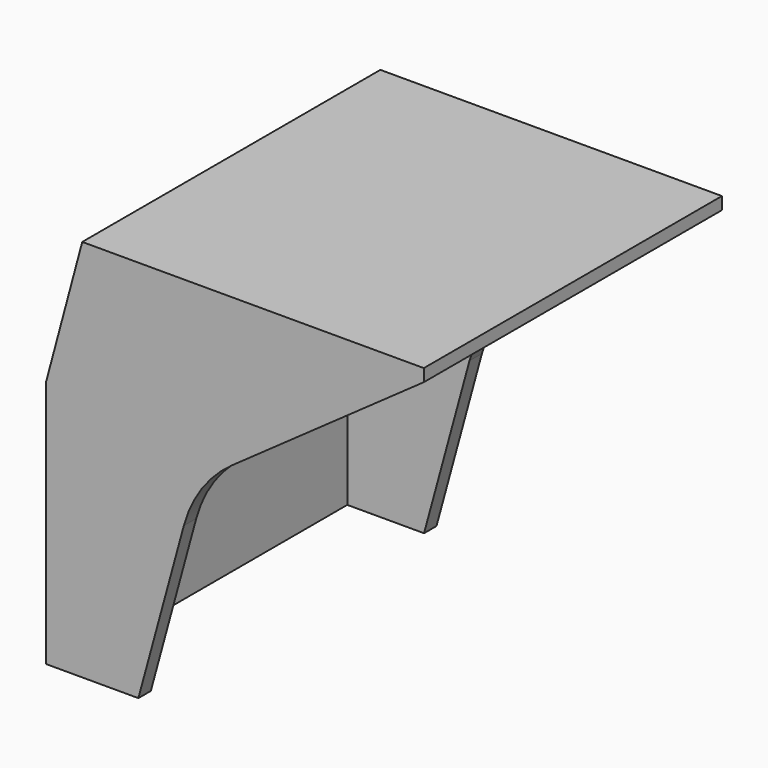
from build123d import *

# Parameters (mm, degrees)
F1_DEPTH  = 120
F2_W      = 85.2778990954
F2_H      = 80
F3_DEPTH  = 98
F6_DEPTH  = 80
F7_W      = 105
F7_H      = 80
F8_DEPTH  = 120
F9_DEPTH  = 15
F10_DEPTH = 30
F11_DEPTH = 15


with BuildPart() as f1:
    # F0 (on Front) → F1 (new body)
    with BuildSketch(Plane.XZ):
        with BuildLine():
            Line((0, 80), (0, 0))
            Line((0, 0), (29.7221009046, 0))
            Line((29.7221009046, 0), (44.3633417849, 53.6774845415))
            ThreePointArc((44.3633417849, 53.6774845415), (50.1903143406, 66.0986305535), (59.871849565, 75.8200683645))
            Line((59.871849565, 75.8200683645), (121.6468570296, 119.466662183))
            Line((121.6468570296, 119.466662183), (121.6468570296, 123.466662183))
            Line((121.6468570296, 123.466662183), (11.6468570296, 123.466662183))
            Line((11.6468570296, 123.466662183), (0, 80))
        make_face()
    extrude(amount=F1_DEPTH)

    # F2 (on face) → F3 (cut)
    with BuildSketch(Plane(origin=(0, 0, 0), x_dir=(1, 0, 0), z_dir=(0, 0, -1))):
        with Locations((72.3610504523, 60)):
            Rectangle(F2_W, F2_H)
        Polygon((5, 100), (5, 60), (5, 20), (29.7221009046, 20), (29.7221009046, 100), align=None)
    extrude(amount=-F3_DEPTH, mode=Mode.SUBTRACT)

    # F5 (on offset) → F6 (cut)
    with BuildSketch(Plane(origin=(-15.1703708686, 0, 4.0648886231), x_dir=(0, -1, 0), z_dir=(-0.9659258263, 0, 0.2588190451))):
        Polygon((115, 79.7740661031), (115, 99.7740661031), (115, 119.7740661031), (35, 119.7740661031), (35, 79.7740661031), align=None)
    extrude(amount=-F6_DEPTH, mode=Mode.SUBTRACT)

    # F7 (on Top) → F8 (cut)
    with BuildSketch(Plane.XY):
        with Locations((68.3294385483, -75)):
            Rectangle(F7_W, F7_H)
    extrude(amount=F8_DEPTH, mode=Mode.SUBTRACT)

    # F9 (cut): a face of the model
    f9_faces = [f1.faces().sort_by_distance(p)[0] for p in [
        (29.9652985241, -20, 58.8911596381),
    ]]
    extrude(f9_faces, amount=-F9_DEPTH, mode=Mode.SUBTRACT)

    # F10 (cut): a face of the model
    f10_faces = [f1.faces().sort_by_distance(p)[0] for p in [
        (60.278784087, -35, 109.488672273),
    ]]
    extrude(f10_faces, amount=-F10_DEPTH, mode=Mode.SUBTRACT)

    # F11 (cut): a face of the model
    f11_faces = [f1.faces().sort_by_distance(p)[0] for p in [
        (10.1941550896, -100, 42.5407610302),
    ]]
    extrude(f11_faces, amount=-F11_DEPTH, mode=Mode.SUBTRACT)


solid = f1.part
